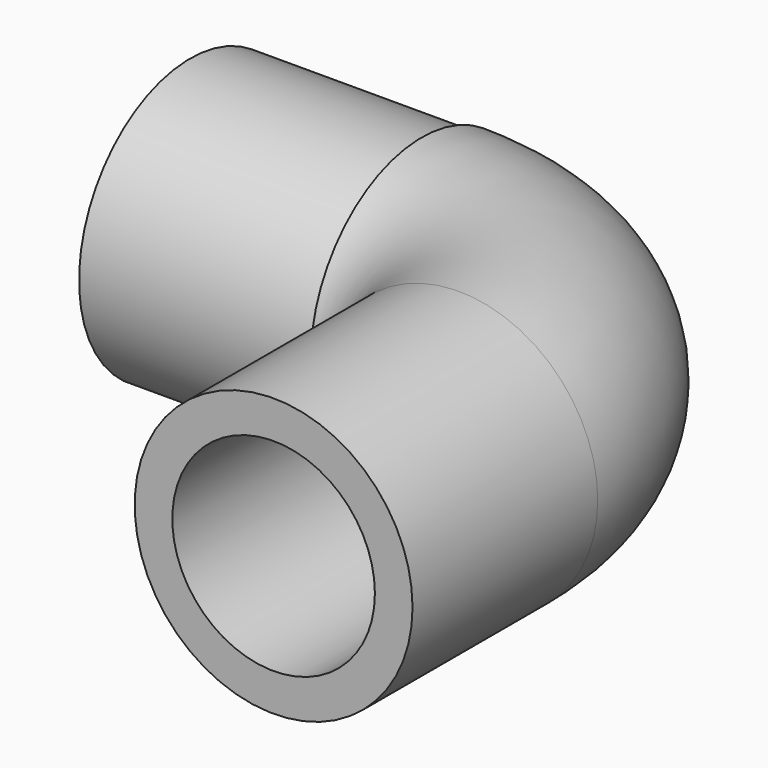
from build123d import *

# Parameters (mm, degrees)
F0_R        = 15.24
F0_R_2      = 11.1125
F2_DEPTH    = 25.4
F1_R        = 15.24
F1_R_2      = 11.1125
F3_DEPTH    = 25.4
F2_FACE_R   = 15.24
F2_FACE_R_2 = 11.1125


with BuildPart() as f2:
    # F0 (on Front) → F2 (new body)
    with BuildSketch(Plane.XZ):
        with Locations((20.32, 0.640698825)):
            Circle(F0_R)
        with Locations((20.32, 0.640698825)):
            Circle(F0_R_2, mode=Mode.SUBTRACT)
    extrude(amount=F2_DEPTH)

    # F5: sweep along a path in F4
    with BuildLine(Plane.XY) as f5_path:
        ThreePointArc((35.4710668325, 0), (25.0818318932, 25.0818318932), (0, 35.4710668325))
    # F2_face (on face) → F5 (sweep)
    with BuildSketch(Plane(origin=(20.32, 0, 0.640698825), x_dir=(1, 0, 0), z_dir=(0, 1, 0))):
        Circle(F2_FACE_R)
        Circle(F2_FACE_R_2, mode=Mode.SUBTRACT)
    sweep(path=f5_path.line)


with BuildPart() as f3:
    # F1 (on Right) → F3 (new body)
    with BuildSketch(Plane.YZ):
        with Locations((20.32, 0)):
            Circle(F1_R)
        with Locations((20.32, 0)):
            Circle(F1_R_2, mode=Mode.SUBTRACT)
    extrude(amount=-F3_DEPTH)


solid = Compound([f2.part, f3.part])
